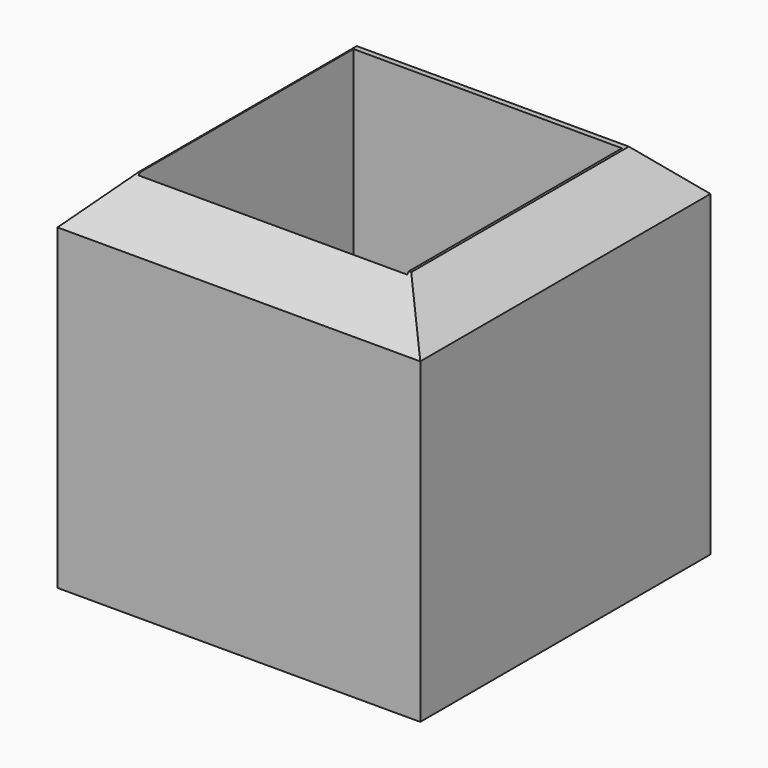
from build123d import *

# Parameters (mm, degrees)
F0_W        = 40
F0_H        = 40
F1_DEPTH    = 40
F2_W        = 29.62
F2_H        = 29.62
F3_DEPTH    = 29.62
F4_T1_DEPTH = 65.7168298797
F4_T3_DEPTH = 65.7168298797


# Not quite as in the source:
# - a fillet or chamfer that OpenCascade refuses, or shapes differently, is made with other operations: its cross-section is extruded or revolved along the edge and cut away or added


with BuildPart() as f1:
    # F0 (on Top) → F1 (new body)
    with BuildSketch(Plane.XY):
        with Locations((20, 20)):
            Rectangle(F0_W, F0_H)
    extrude(amount=F1_DEPTH)

    # F2 (on face) → F3 (cut)
    with BuildSketch(Plane.XY.offset(40)):
        with Locations((19.9230909348, 19.5811167631)):
            Rectangle(F2_W, F2_H)
    extrude(amount=-F3_DEPTH, mode=Mode.SUBTRACT)

    # F4: chamfer of 5 on 4 edges, made by hand

    # F4_s2 → F4_t1 (cut)
    with BuildSketch(Plane.YZ.offset(-12.8584149398)):
        Polygon((0, 35), (5, 40), (0, 40), align=None)
        Polygon((40, 35), (35, 40), (40, 40), align=None)
    extrude(amount=F4_T1_DEPTH, mode=Mode.SUBTRACT)

    # F4_s4 → F4_t3 (cut)
    with BuildSketch(Plane.XZ.offset(-52.8584149398)):
        Polygon((35, 40), (40, 35), (40, 40), align=None)
        Polygon((0, 35), (5, 40), (0, 40), align=None)
    extrude(amount=F4_T3_DEPTH, mode=Mode.SUBTRACT)


solid = f1.part
